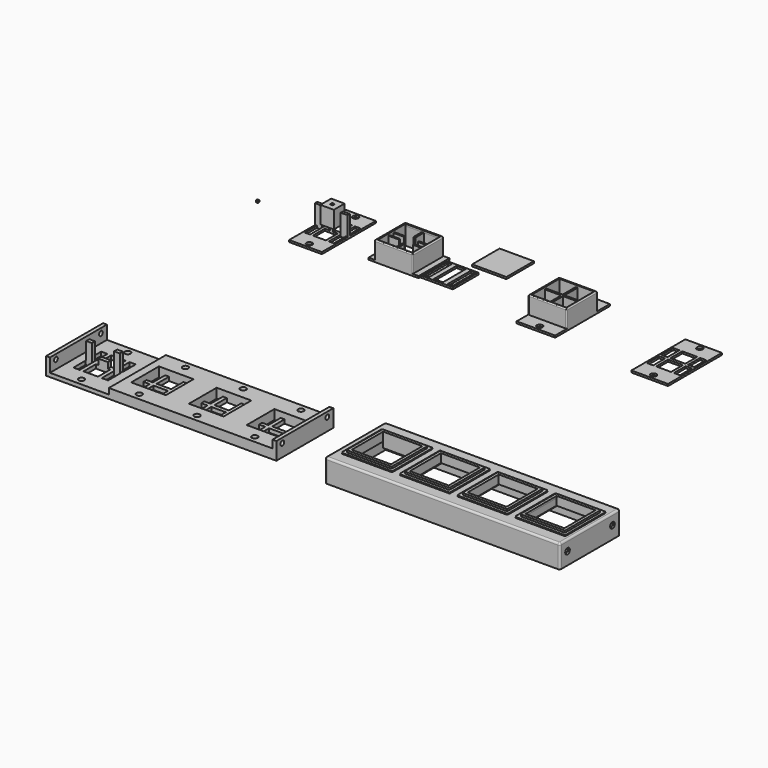
from build123d import *

# Parameters (mm, degrees)
F0_W          = 20
F0_H          = 20
F1_DEPTH      = 10
F2_T          = -1
F4_DEPTH      = 9
F5_W          = 20
F5_H          = 8
F5_R          = 1.5
F6_DEPTH      = 1
F7_W          = 19
F7_H          = 19
F7_H_2        = 8
F7_R          = 1.5
F8_DEPTH      = 1
F9_W          = 20
F9_H          = 20
F10_DEPTH     = 10
F11_W         = 3
F11_H         = 20
F11_W_2       = 20
F12_DEPTH     = 0.95
F13_T         = 1
F13_T3_DEPTH  = 22
F14_W         = 8.5
F14_H         = 0.8
F15_DEPTH     = 9
F17_DEPTH     = 9
F18_W         = 17
F18_H         = 8
F18_R         = 1.5
F18_H_2       = 19
F19_DEPTH     = 1
F20_W         = 1.5
F20_H         = 1.5
F21_DEPTH     = 3
F22_W         = 7
F22_H         = 7
F22_W_2       = 1.5
F22_H_2       = 1.5
F23_DEPTH     = 9
F24_W         = 1
F24_H         = 1
F25_DEPTH     = 1
F27_DEPTH     = 10
F28_W         = 0.9
F28_H         = 14.7
F28_W_2       = 2.5
F28_H_2       = 0.8
F28_H_3       = 6
F28_H_4       = 1.1
F29_DEPTH     = 1
F30_W         = 117
F30_H         = 37
F30_R         = 1.5
F31_DEPTH     = 1
F32_W         = 122
F32_H         = 39.2
F32_W_2       = 20.4
F32_H_2       = 20.4
F32_W_3       = 20.2
F32_H_3       = 20.2
F33_DEPTH     = 11
F34_W         = 120
F34_H         = 37.2
F35_DEPTH     = 8
F36_W         = 4
F36_H         = 18
F37_DEPTH     = 3
F39_W         = 3
F39_H         = 2
F40_DEPTH     = 9
F41_W         = 5
F41_H         = 2
F42_DEPTH     = 3
F43_R         = 1
F44_R         = 0.5
F44_2_R       = 0.5
F38_R         = 1.5
F45_DEPTH     = 3
F46_DEPTH     = 2
F47_W         = 2
F47_H         = 37
F48_DEPTH     = 7
F49_W         = 20.4
F49_H         = 8.4
F50_DEPTH     = 3
F51_R         = 1.5
F52_DEPTH     = 3
F54_R         = 1.5
F55_DEPTH     = 2
F56_W         = 3
F56_H         = 37.2
F57_DEPTH     = 1
F58_DEPTH     = 1
F59_W         = 2
F59_H         = 37
F60_DEPTH     = 4
F53_R         = 1.2
F61_DEPTH     = 269.2358512024
F62_DEPTH     = 3
F63_DEPTH     = 5
F46_FACE2_W   = 119
F46_FACE2_H   = 37
F46_FACE2_R   = 1.5
F46_FACE2_W_2 = 3.25
F46_FACE2_H_2 = 8
F46_FACE2_W_3 = 7.5
F64_DEPTH     = 1
F65_DEPTH     = 1
F66_DEPTH     = 2
F67_DEPTH     = 0.05
F68_W         = 20.4
F68_H         = 3
F68_W_2       = 20.2
F68_H_2       = 3.1
F69_DEPTH     = 0.5
F70_W         = 20.4
F70_H         = 1.5
F70_W_2       = 20.2
F71_DEPTH     = 1
F72_R         = 0.5
F73_W         = 18
F73_H         = 17.9999990673
F74_DEPTH     = 1
F75_W         = 17.8
F75_H         = 17.8
F76_DEPTH     = 1
F77_W         = 18
F77_H         = 18
F78_DEPTH     = 1


# Not quite as in the source:
# - a shell that OpenCascade refuses in one call is made with other operations: the cavity is built on its own and cut out
# - a feature names something its author has since deleted; it is built from what else it names


with BuildPart() as f1:
    # F0 (on Top) → F1 (new body)
    with BuildSketch(Plane.XY):
        Rectangle(F0_W, F0_H)
    extrude(amount=F1_DEPTH)

    # F2
    f2_openings = [f1.faces().sort_by_distance(p)[0] for p in [
        (0, 0, 0),
    ]]
    offset(amount=F2_T, openings=f2_openings)

    # F3 (on Top) → F4 (join)
    with BuildSketch(Plane.XY):
        Polygon((-0.5, -9), (0.5, -9), (0.5, -0.5), (9, -0.5), (9, 0.5), (0.5, 0.5), (0.5, 9), (-0.5, 9), (-0.5, 0.5), (-9, 0.5), (-9, -0.5), (-0.5, -0.5), align=None)
    extrude(amount=F4_DEPTH)

    # F5 (on Top) → F6 (join)
    with BuildSketch(Plane.XY):
        with Locations((0, -13.5)):
            Rectangle(F5_W, F5_H)
        with Locations((0, -15)):
            Circle(F5_R, mode=Mode.SUBTRACT)
        with Locations((0, 14)):
            Rectangle(F5_W, F5_H)
        with Locations((0, 15)):
            Circle(F5_R, mode=Mode.SUBTRACT)
    extrude(amount=F6_DEPTH)

    # F44
    f44_edges = [f1.edges().sort_by_distance(p)[0] for p in [
        (-10, -10, 5.5),
        (0, -10, 10),
        (10, -10, 5.5),
        (-10, 0, 10),
        (-10, 10, 5.5),
        (0, 10, 10),
        (10, 10, 5.5),
        (10, 0, 10),
    ]]
    fillet(f44_edges, radius=F44_R)

    # F77 (on face) → F78 (cut)
    with BuildSketch(Plane.XY.offset(10)):
        Rectangle(F77_W, F77_H)
    extrude(amount=-F78_DEPTH, mode=Mode.SUBTRACT)


with BuildPart() as f8:
    # F7 (on Top) → F8 (new body)
    with BuildSketch(Plane.XY):
        with Locations((62.8032131791, -4.6075988114)):
            Rectangle(F7_W, F7_H)
        Polygon((54.3032131791, -3.8575988114), (54.3032131791, 3.8924011886), (57.4282131791, 3.8924011886), (58.9282131791, 3.8924011886), (66.6782131791, 3.8924011886), (68.1782131791, 3.8924011886), (71.3032131791, 3.8924011886), (71.3032131791, -3.8575988114), (71.3032131791, -5.3575988114), (71.3032131791, -13.1075988114), (68.1782131791, -13.1075988114), (66.6782131791, -13.1075988114), (58.9282131791, -13.1075988114), (57.4282131791, -13.1075988114), (54.3032131791, -13.1075988114), (54.3032131791, -5.3575988114), align=None, mode=Mode.SUBTRACT)
        with Locations((62.8032131791, 8.8924011886)):
            Rectangle(F7_W, F7_H_2)
        with Locations((62.8032131791, 10.3924011886)):
            Circle(F7_R, mode=Mode.SUBTRACT)
        with Locations((62.8032131791, -18.1075988114)):
            Rectangle(F7_W, F7_H_2)
        with Locations((62.8032131791, -19.6075988114)):
            Circle(F7_R, mode=Mode.SUBTRACT)
        Polygon((58.9282131791, 3.8924011886), (57.4282131791, 3.8924011886), (57.4282131791, -3.8575988114), (54.3032131791, -3.8575988114), (54.3032131791, -5.3575988114), (57.4282131791, -5.3575988114), (57.4282131791, -13.1075988114), (58.9282131791, -13.1075988114), (58.9282131791, -5.3575988114), (66.6782131791, -5.3575988114), (66.6782131791, -13.1075988114), (68.1782131791, -13.1075988114), (68.1782131791, -5.3575988114), (71.3032131791, -5.3575988114), (71.3032131791, -3.8575988114), (68.1782131791, -3.8575988114), (68.1782131791, 3.8924011886), (66.6782131791, 3.8924011886), (66.6782131791, -3.8575988114), (58.9282131791, -3.8575988114), align=None)
    extrude(amount=F8_DEPTH)


with BuildPart() as f10:
    # F9 (on Top) → F10 (new body)
    with BuildSketch(Plane.XY):
        with Locations((-78.8846665621, -1.3073290847)):
            Rectangle(F9_W, F9_H)
    extrude(amount=F10_DEPTH)

    # F11 (on face) → F12 (join)
    with BuildSketch(Plane(origin=(0, 0, 0), x_dir=(1, 0, 0), z_dir=(0, 0, -1))):
        with Locations((-90.3846665621, 1.3073290847)):
            Rectangle(F11_W, F11_H)
        with Locations((-78.8846665621, 1.3073290847)):
            Rectangle(F11_W_2, F11_H)
        with Locations((-67.3846665621, 1.3073290847)):
            Rectangle(F11_W, F11_H)
    extrude(amount=-F12_DEPTH)

    # F13: shell of thickness 1, made by hand


with BuildPart() as f13_core1:
    # F13_t2: copy of F10
    add(f10.part)

    # the walls: a layer under each face that stays
    f13_faces = [f13_core1.faces().sort_by_distance(p)[0] for p in [
        (-78.8846665621, 8.6926709153, 5),
        (-91.8846665621, -1.3073290847, 0.475),
        (-78.8846665621, -11.3073290847, 5),
        (-90.3846665621, -1.3073290847, 0.95),
        (-88.8846665621, -1.3073290847, 5.475),
        (-78.8846665621, -1.3073290847, 10),
        (-68.8846665621, -1.3073290847, 5.475),
        (-67.3846665621, -1.3073290847, 0.95),
        (-65.8846665621, -1.3073290847, 0.475),
    ]]
    thicken(f13_faces, amount=-F13_T, mode=Mode.SUBTRACT)

    # F13_s4 → F13_t3 (cut)
    with BuildSketch(Plane.XZ.offset(-9.6926709153)):
        Polygon((-88.8946665621, 0.96), (-88.8846665621, -0.05), (-87.8846665621, -0.05), (-87.8846665621, 0.95), align=None)
        Polygon((-68.8746665621, 0.96), (-69.8846665621, 0.95), (-69.8846665621, -0.05), (-68.8846665621, -0.05), align=None)
    extrude(amount=F13_T3_DEPTH, mode=Mode.SUBTRACT)


with BuildPart() as f10_1:
    add(f10.part)

    # what is left inside the walls is the cavity
    f13_cavity = [f13_core1.part.solids().sort_by_distance(p)[0] for p in [
        (-78.884667, -4.307329, 0.01),
    ]]
    add(f13_cavity, mode=Mode.SUBTRACT)

    # F14 (on Top) → F15 (join)
    with BuildSketch(Plane.XY):
        Polygon((-78.3846665621, 7.6926709153), (-79.3846665621, 7.6926709153), (-79.3846665621, 0.6926709153), (-79.3846665621, -0.1073290847), (-79.3846665621, -2.5073290847), (-79.3846665621, -3.3073290847), (-79.3846665621, -10.3073290847), (-78.3846665621, -10.3073290847), (-78.3846665621, -3.3073290847), (-78.3846665621, -2.5073290847), (-78.3846665621, -0.1073290847), (-78.3846665621, 0.6926709153), align=None)
        with Locations((-83.6346665621, -2.9073290847)):
            Rectangle(F14_W, F14_H)
        with Locations((-83.6346665621, 0.2926709153)):
            Rectangle(F14_W, F14_H)
        with Locations((-74.1346665621, 0.2926709153)):
            Rectangle(F14_W, F14_H)
        with Locations((-74.1346665621, -2.9073290847)):
            Rectangle(F14_W, F14_H)
    extrude(amount=F15_DEPTH)

    # F16 (on face) → F17 (cut)
    with BuildSketch(Plane(origin=(0, 0, 0), x_dir=(1, 0, 0), z_dir=(0, 0, -1))):
        Polygon((-79.3846665621, -2.2926709153), (-78.3846665621, -2.2926709153), (-78.3846665621, -0.6926709153), (-75.2846665621, -0.6926709153), (-75.2846665621, 0.1073290847), (-78.3846665621, 0.1073290847), (-78.3846665621, 2.5073290847), (-75.2846665621, 2.5073290847), (-75.2846665621, 3.3073290847), (-78.3846665621, 3.3073290847), (-78.3846665621, 4.9073290847), (-79.3846665621, 4.9073290847), (-79.3846665621, 3.3073290847), (-82.4846665621, 3.3073290847), (-82.4846665621, 2.5073290847), (-79.3846665621, 2.5073290847), (-79.3846665621, 0.1073290847), (-82.4846665621, 0.1073290847), (-82.4846665621, -0.6926709153), (-79.3846665621, -0.6926709153), align=None)
    extrude(amount=-F17_DEPTH, mode=Mode.SUBTRACT)

    # F44#2
    f44_2_edges = [f10_1.edges().sort_by_distance(p)[0] for p in [
        (-68.884667, -11.307329, 5.475),
        (-78.884667, -11.307329, 10),
        (-68.884667, -1.307329, 10),
        (-68.884667, 8.692671, 5.475),
        (-78.884667, 8.692671, 10),
        (-88.884667, 8.692671, 5.475),
        (-88.884667, -1.307329, 10),
        (-88.884667, -11.307329, 5.475),
    ]]
    fillet(f44_2_edges, radius=F44_2_R)

    # F67 (add): faces of the model
    f67_faces = [f10_1.faces().sort_by_distance(p)[0] for p in [
        (-90.3817894545, -1.3073290847, 0.95),
        (-67.3875436696, -1.3073290847, 0.95),
    ]]
    extrude(f67_faces, amount=F67_DEPTH)

    # F73 (on face) → F74 (cut)
    with BuildSketch(Plane.XY.offset(10)):
        with Locations((-78.8846665621, -1.3073295511)):
            Rectangle(F73_W, F73_H)
    extrude(amount=-F74_DEPTH, mode=Mode.SUBTRACT)


with BuildPart() as f19:
    # F18 (on Top) → F19 (new body)
    with BuildSketch(Plane.XY):
        with Locations((-118.1940851788, 11.6607970074)):
            Rectangle(F18_W, F18_H)
        with Locations((-118.1940851788, 13.1607970074)):
            Circle(F18_R, mode=Mode.SUBTRACT)
        with Locations((-118.1940851788, -15.3392029926)):
            Rectangle(F18_W, F18_H)
        with Locations((-118.1940851788, -16.8392029926)):
            Circle(F18_R, mode=Mode.SUBTRACT)
        with Locations((-118.1940851788, -1.8392029926)):
            Rectangle(F18_W, F18_H_2)
        Polygon((-125.6940851788, -1.0892029926), (-125.6940851788, 6.6607970074), (-123.0690851788, 6.6607970074), (-121.5690851788, 6.6607970074), (-114.8190851788, 6.6607970074), (-113.3190851788, 6.6607970074), (-110.6940851788, 6.6607970074), (-110.6940851788, -1.0892029926), (-110.6940851788, -2.5892029926), (-110.6940851788, -10.3392029926), (-113.3190851788, -10.3392029926), (-114.8190851788, -10.3392029926), (-121.5690851788, -10.3392029926), (-123.0690851788, -10.3392029926), (-125.6940851788, -10.3392029926), (-125.6940851788, -2.5892029926), align=None, mode=Mode.SUBTRACT)
        Polygon((-121.5690851788, 6.6607970074), (-123.0690851788, 6.6607970074), (-123.0690851788, -1.0892029926), (-125.6940851788, -1.0892029926), (-125.6940851788, -2.5892029926), (-123.0690851788, -2.5892029926), (-123.0690851788, -10.3392029926), (-121.5690851788, -10.3392029926), (-121.5690851788, -2.5892029926), (-114.8190851788, -2.5892029926), (-114.8190851788, -10.3392029926), (-113.3190851788, -10.3392029926), (-113.3190851788, -2.5892029926), (-110.6940851788, -2.5892029926), (-110.6940851788, -1.0892029926), (-113.3190851788, -1.0892029926), (-113.3190851788, 6.6607970074), (-114.8190851788, 6.6607970074), (-114.8190851788, -1.0892029926), (-121.5690851788, -1.0892029926), align=None)
    extrude(amount=F19_DEPTH)

    # F20 (on face) → F21 (join)
    with BuildSketch(Plane.XY.offset(1)):
        with Locations((-118.1940851788, -1.8392029926)):
            Rectangle(F20_W, F20_H)
    extrude(amount=F21_DEPTH)

    # F26 (on face) → F27 (join)
    with BuildSketch(Plane.XY.offset(1)):
        Polygon((-109.6940851788, -2.5892029926), (-109.6940851788, -1.0892029926), (-110.6940851788, -1.0892029926), (-113.3190851788, -1.0892029926), (-113.3190851788, -2.5892029926), (-110.6940851788, -2.5892029926), align=None)
        Polygon((-125.6940851788, -1.0892029926), (-126.6940851788, -1.0892029926), (-126.6940851788, -2.5892029926), (-125.6940851788, -2.5892029926), (-123.0690851788, -2.5892029926), (-123.0690851788, -1.0892029926), align=None)
    extrude(amount=F27_DEPTH)


with BuildPart() as f23:
    # F22 (on face) → F23 (new body)
    with BuildSketch(Plane.XY.offset(4)):
        with Locations((-118.1940851788, -1.8392029926)):
            Rectangle(F22_W, F22_H)
        with Locations((-118.1940851788, -1.8392029926)):
            Rectangle(F22_W_2, F22_H_2, mode=Mode.SUBTRACT)
    extrude(amount=F23_DEPTH)


with BuildPart() as f25:
    # F24 (on Top) → F25 (new body)
    with BuildSketch(Plane.XY):
        with Locations((-158.5527062416, 0)):
            Rectangle(F24_W, F24_H)
    extrude(amount=F25_DEPTH)


with BuildPart() as f29:
    # F28 (on Top) → F29 (new body)
    with BuildSketch(Plane.XY):
        Polygon((-64.4713718057, -9.4157041669), (-65.3713718057, -9.4157041669), (-65.3713718057, -10.3157041669), (-54.7713718057, -10.3157041669), (-52.2713718057, -10.3157041669), (-48.8713718057, -10.3157041669), (-48.8713718057, -9.4157041669), (-49.7713718057, -9.4157041669), (-52.2713718057, -9.4157041669), (-54.7713718057, -9.4157041669), (-59.4713718057, -9.4157041669), (-61.9713718057, -9.4157041669), align=None)
        with Locations((-64.9213718057, -2.0657041669)):
            Rectangle(F28_W, F28_H)
        Polygon((-48.8713718057, 6.1842958331), (-65.3713718057, 6.1842958331), (-65.3713718057, 5.2842958331), (-64.4713718057, 5.2842958331), (-61.9713718057, 5.2842958331), (-59.4713718057, 5.2842958331), (-54.7713718057, 5.2842958331), (-52.2713718057, 5.2842958331), (-49.7713718057, 5.2842958331), (-48.8713718057, 5.2842958331), align=None)
        with Locations((-49.3213718057, -2.0657041669)):
            Rectangle(F28_W, F28_H)
        with Locations((-53.5213718057, 4.8842958331)):
            Rectangle(F28_W_2, F28_H_2)
        with Locations((-53.5213718057, 1.4842958331)):
            Rectangle(F28_W_2, F28_H_3)
        with Locations((-53.5213718057, -2.0657041669)):
            Rectangle(F28_W_2, F28_H_4)
        with Locations((-53.5213718057, -5.6157041669)):
            Rectangle(F28_W_2, F28_H_3)
        with Locations((-53.5213718057, -9.0157041669)):
            Rectangle(F28_W_2, F28_H_2)
        with Locations((-60.7213718057, 4.8842958331)):
            Rectangle(F28_W_2, F28_H_2)
        with Locations((-60.7213718057, 1.4842958331)):
            Rectangle(F28_W_2, F28_H_3)
        with Locations((-60.7213718057, -2.0657041669)):
            Rectangle(F28_W_2, F28_H_4)
        with Locations((-60.7213718057, -5.6157041669)):
            Rectangle(F28_W_2, F28_H_3)
        with Locations((-60.7213718057, -9.0157041669)):
            Rectangle(F28_W_2, F28_H_2)
    extrude(amount=F29_DEPTH)


with BuildPart() as f31:
    # F30 (on Top) → F31 (new body)
    with BuildSketch(Plane.XY):
        with Locations((-71.0754835367, -152.5580135584)):
            Rectangle(F30_W, F30_H)
        with Locations((-115.9754835367, -167.5580135584)):
            Circle(F30_R, mode=Mode.SUBTRACT)
        with Locations((-85.9754835367, -167.5580135584)):
            Circle(F30_R, mode=Mode.SUBTRACT)
        Polygon((-124.9754835367, -151.5580135584), (-124.9754835367, -143.5580135584), (-121.7254835367, -143.5580135584), (-119.7254835367, -143.5580135584), (-112.2254835367, -143.5580135584), (-110.2254835367, -143.5580135584), (-106.9754835367, -143.5580135584), (-106.9754835367, -151.5580135584), (-106.9754835367, -153.5580135584), (-106.9754835367, -161.5580135584), (-110.2254835367, -161.5580135584), (-112.2254835367, -161.5580135584), (-119.7254835367, -161.5580135584), (-121.7254835367, -161.5580135584), (-124.9754835367, -161.5580135584), (-124.9754835367, -153.5580135584), align=None, mode=Mode.SUBTRACT)
        Polygon((-94.9754835367, -151.5580135584), (-94.9754835367, -143.5580135584), (-91.7254835367, -143.5580135584), (-89.7254835367, -143.5580135584), (-82.2254835367, -143.5580135584), (-80.2254835367, -143.5580135584), (-76.9754835367, -143.5580135584), (-76.9754835367, -151.5580135584), (-76.9754835367, -153.5580135584), (-76.9754835367, -161.5580135584), (-80.2254835367, -161.5580135584), (-82.2254835367, -161.5580135584), (-89.7254835367, -161.5580135584), (-91.7254835367, -161.5580135584), (-94.9754835367, -161.5580135584), (-94.9754835367, -153.5580135584), align=None, mode=Mode.SUBTRACT)
        with Locations((-55.9754835367, -167.5580135584)):
            Circle(F30_R, mode=Mode.SUBTRACT)
        with Locations((-25.9754835367, -167.5580135584)):
            Circle(F30_R, mode=Mode.SUBTRACT)
        Polygon((-64.9754835367, -151.5580135584), (-64.9754835367, -143.5580135584), (-61.7254835367, -143.5580135584), (-59.7254835367, -143.5580135584), (-52.2254835367, -143.5580135584), (-50.2254835367, -143.5580135584), (-46.9754835367, -143.5580135584), (-46.9754835367, -151.5580135584), (-46.9754835367, -153.5580135584), (-46.9754835367, -161.5580135584), (-47.9754835367, -161.5580135584), (-50.2254835367, -161.5580135584), (-52.2254835367, -161.5580135584), (-59.7254835367, -161.5580135584), (-61.7254835367, -161.5580135584), (-64.9754835367, -161.5580135584), (-64.9754835367, -153.5580135584), align=None, mode=Mode.SUBTRACT)
        Polygon((-34.9754835367, -151.5580135584), (-34.9754835367, -143.5580135584), (-31.7254835367, -143.5580135584), (-29.7254835367, -143.5580135584), (-22.2254835367, -143.5580135584), (-20.2254835367, -143.5580135584), (-16.9754835367, -143.5580135584), (-16.9754835367, -151.5580135584), (-16.9754835367, -153.5580135584), (-16.9754835367, -161.5580135584), (-17.9754835367, -161.5580135584), (-20.2254835367, -161.5580135584), (-22.2254835367, -161.5580135584), (-29.7254835367, -161.5580135584), (-31.7254835367, -161.5580135584), (-34.9754835367, -161.5580135584), (-34.9754835367, -153.5580135584), align=None, mode=Mode.SUBTRACT)
        with Locations((-115.9754835367, -137.5580135584)):
            Circle(F30_R, mode=Mode.SUBTRACT)
        with Locations((-85.9754835367, -137.5580135584)):
            Circle(F30_R, mode=Mode.SUBTRACT)
        with Locations((-55.9754835367, -137.5580135584)):
            Circle(F30_R, mode=Mode.SUBTRACT)
        with Locations((-25.9754835367, -137.5580135584)):
            Circle(F30_R, mode=Mode.SUBTRACT)
        Polygon((-119.7254835367, -143.5580135584), (-121.7254835367, -143.5580135584), (-121.7254835367, -151.5580135584), (-124.9754835367, -151.5580135584), (-124.9754835367, -153.5580135584), (-121.7254835367, -153.5580135584), (-121.7254835367, -161.5580135584), (-119.7254835367, -161.5580135584), (-119.7254835367, -153.5580135584), (-112.2254835367, -153.5580135584), (-112.2254835367, -161.5580135584), (-110.2254835367, -161.5580135584), (-110.2254835367, -153.5580135584), (-106.9754835367, -153.5580135584), (-106.9754835367, -151.5580135584), (-110.2254835367, -151.5580135584), (-110.2254835367, -143.5580135584), (-112.2254835367, -143.5580135584), (-112.2254835367, -151.5580135584), (-119.7254835367, -151.5580135584), align=None)
        Polygon((-89.7254835367, -143.5580135584), (-91.7254835367, -143.5580135584), (-91.7254835367, -151.5580135584), (-94.9754835367, -151.5580135584), (-94.9754835367, -153.5580135584), (-91.7254835367, -153.5580135584), (-91.7254835367, -161.5580135584), (-89.7254835367, -161.5580135584), (-89.7254835367, -153.5580135584), (-82.2254835367, -153.5580135584), (-82.2254835367, -161.5580135584), (-80.2254835367, -161.5580135584), (-80.2254835367, -153.5580135584), (-76.9754835367, -153.5580135584), (-76.9754835367, -151.5580135584), (-80.2254835367, -151.5580135584), (-80.2254835367, -143.5580135584), (-82.2254835367, -143.5580135584), (-82.2254835367, -151.5580135584), (-89.7254835367, -151.5580135584), align=None)
        Polygon((-59.7254835367, -143.5580135584), (-61.7254835367, -143.5580135584), (-61.7254835367, -151.5580135584), (-64.9754835367, -151.5580135584), (-64.9754835367, -153.5580135584), (-61.7254835367, -153.5580135584), (-61.7254835367, -161.5580135584), (-59.7254835367, -161.5580135584), (-59.7254835367, -153.5580135584), (-52.2254835367, -153.5580135584), (-52.2254835367, -161.5580135584), (-50.2254835367, -161.5580135584), (-50.2254835367, -153.5580135584), (-46.9754835367, -153.5580135584), (-46.9754835367, -151.5580135584), (-50.2254835367, -151.5580135584), (-50.2254835367, -143.5580135584), (-52.2254835367, -143.5580135584), (-52.2254835367, -151.5580135584), (-59.7254835367, -151.5580135584), align=None)
        Polygon((-29.7254835367, -143.5580135584), (-31.7254835367, -143.5580135584), (-31.7254835367, -151.5580135584), (-34.9754835367, -151.5580135584), (-34.9754835367, -153.5580135584), (-31.7254835367, -153.5580135584), (-31.7254835367, -161.5580135584), (-29.7254835367, -161.5580135584), (-29.7254835367, -153.5580135584), (-22.2254835367, -153.5580135584), (-22.2254835367, -161.5580135584), (-20.2254835367, -161.5580135584), (-20.2254835367, -153.5580135584), (-16.9754835367, -153.5580135584), (-16.9754835367, -151.5580135584), (-20.2254835367, -151.5580135584), (-20.2254835367, -143.5580135584), (-22.2254835367, -143.5580135584), (-22.2254835367, -151.5580135584), (-29.7254835367, -151.5580135584), align=None)
    extrude(amount=F31_DEPTH)

    # F36 (on face) → F37 (join)
    with BuildSketch(Plane.XY.offset(1)):
        with Locations((-96.9754835367, -152.5580135584)):
            Rectangle(F36_W, F36_H)
        with Locations((-74.9754835367, -152.5580135584)):
            Rectangle(F36_W, F36_H)
        with Locations((-66.9754835367, -152.5580135584)):
            Rectangle(F36_W, F36_H)
        with Locations((-44.9754835367, -152.5580135584)):
            Rectangle(F36_W, F36_H)
        with Locations((-36.9754835367, -152.5580135584)):
            Rectangle(F36_W, F36_H)
        with Locations((-14.9754835367, -152.5580135584)):
            Rectangle(F36_W, F36_H)
    extrude(amount=F37_DEPTH)

    # F39 (on face) → F40 (join)
    with BuildSketch(Plane.XY.offset(1)):
        with Locations((-123.2254835367, -152.5580135584)):
            Rectangle(F39_W, F39_H)
        with Locations((-108.7254835367, -152.5580135584)):
            Rectangle(F39_W, F39_H)
    extrude(amount=F40_DEPTH)

    # F41 (on face) → F42 (join)
    with BuildSketch(Plane.XY.offset(1)):
        with Locations((-115.9754835367, -152.5580135584)):
            Rectangle(F41_W, F41_H)
    extrude(amount=F42_DEPTH)

    # F38 (on face) → F45 (join)
    with BuildSketch(Plane.XY.offset(1)):
        Polygon((-98.9754835367, -134.0580135584), (-98.9754835367, -143.5580135584), (-94.9754835367, -143.5580135584), (-91.7254835367, -143.5580135584), (-89.7254835367, -143.5580135584), (-82.2254835367, -143.5580135584), (-80.2254835367, -143.5580135584), (-76.9754835367, -143.5580135584), (-72.9754835367, -143.5580135584), (-72.9754835367, -134.0580135584), align=None)
        with Locations((-85.9754835367, -137.5580135584)):
            Circle(F38_R, mode=Mode.SUBTRACT)
        Polygon((-94.9754835367, -161.5580135584), (-98.9754835367, -161.5580135584), (-98.9754835367, -171.0580135584), (-72.9754835367, -171.0580135584), (-72.9754835367, -161.5580135584), (-76.9754835367, -161.5580135584), (-80.2254835367, -161.5580135584), (-82.2254835367, -161.5580135584), (-89.7254835367, -161.5580135584), (-91.7254835367, -161.5580135584), align=None)
        with Locations((-85.9754835367, -167.5580135584)):
            Circle(F38_R, mode=Mode.SUBTRACT)
        Polygon((-68.9754835367, -161.5580135584), (-68.9754835367, -171.0580135584), (-42.9754835367, -171.0580135584), (-42.9754835367, -161.5580135584), (-46.9754835367, -161.5580135584), (-50.2254835367, -161.5580135584), (-52.2254835367, -161.5580135584), (-59.7254835367, -161.5580135584), (-61.7254835367, -161.5580135584), (-64.9754835367, -161.5580135584), align=None)
        with Locations((-55.9754835367, -167.5580135584)):
            Circle(F38_R, mode=Mode.SUBTRACT)
        Polygon((-42.9754835367, -134.0580135584), (-68.9754835367, -134.0580135584), (-68.9754835367, -143.5580135584), (-64.9754835367, -143.5580135584), (-61.7254835367, -143.5580135584), (-59.7254835367, -143.5580135584), (-52.2254835367, -143.5580135584), (-50.2254835367, -143.5580135584), (-46.9754835367, -143.5580135584), (-42.9754835367, -143.5580135584), align=None)
        with Locations((-55.9754835367, -137.5580135584)):
            Circle(F38_R, mode=Mode.SUBTRACT)
        Polygon((-12.9754835367, -134.0580135584), (-38.9754835367, -134.0580135584), (-38.9754835367, -143.5580135584), (-34.9754835367, -143.5580135584), (-31.7254835367, -143.5580135584), (-29.7254835367, -143.5580135584), (-22.2254835367, -143.5580135584), (-20.2254835367, -143.5580135584), (-16.9754835367, -143.5580135584), (-12.9754835367, -143.5580135584), align=None)
        with Locations((-25.9754835367, -137.5580135584)):
            Circle(F38_R, mode=Mode.SUBTRACT)
        Polygon((-38.9754835367, -161.5580135584), (-38.9754835367, -171.0580135584), (-12.9754835367, -171.0580135584), (-12.9754835367, -161.5580135584), (-16.9754835367, -161.5580135584), (-20.2254835367, -161.5580135584), (-22.2254835367, -161.5580135584), (-29.7254835367, -161.5580135584), (-31.7254835367, -161.5580135584), (-34.9754835367, -161.5580135584), align=None)
        with Locations((-25.9754835367, -167.5580135584)):
            Circle(F38_R, mode=Mode.SUBTRACT)
    extrude(amount=F45_DEPTH)

    # F46 (add): a face of the model
    f46_faces = [f31.faces().sort_by_distance(p)[0] for p in [
        (-129.5754835367, -152.5580135584, 0.5),
    ]]
    extrude(f46_faces, amount=F46_DEPTH)

    # F47 (on face) → F48 (join)
    with BuildSketch(Plane.XY.offset(1)):
        with Locations((-130.5754835367, -152.5580135584)):
            Rectangle(F47_W, F47_H)
    extrude(amount=F48_DEPTH)

    # F58 (add): a face of the model
    f58_faces = [f31.faces().sort_by_distance(p)[0] for p in [
        (-12.9754835367, -152.5580135584, 2.5),
    ]]
    extrude(f58_faces, amount=F58_DEPTH)

    # F59 (on face) → F60 (join)
    with BuildSketch(Plane.XY.offset(4)):
        with Locations((-12.9754835367, -152.5580135584)):
            Rectangle(F59_W, F59_H)
    extrude(amount=F60_DEPTH)

    # F53 (on face) → F61 (cut, through all)
    with BuildSketch(Plane(origin=(-131.5754835367, 0, 0), x_dir=(0, -1, 0), z_dir=(-1, 0, 0))):
        with Locations((137.9580135584, 5.5)):
            Circle(F53_R)
        with Locations((167.1580135584, 5.5)):
            Circle(F53_R)
    extrude(amount=-F61_DEPTH, mode=Mode.SUBTRACT)

    # F63 (add): faces of the model
    f63_faces = [f31.faces().sort_by_distance(p)[0] for p in [
        (-72.9754835367, -152.5580135584, 2.5),
        (-42.9754835367, -152.5580135584, 2.5),
    ]]
    extrude(f63_faces, amount=F63_DEPTH)

    # F30 (on Top) + F46_face2 (on face) → F64 (join)
    with BuildSketch(Plane.XY):
        with Locations((-71.0754835367, -152.5580135584)):
            Rectangle(F30_W, F30_H)
        with Locations((-115.9754835367, -167.5580135584)):
            Circle(F30_R, mode=Mode.SUBTRACT)
        with Locations((-85.9754835367, -167.5580135584)):
            Circle(F30_R, mode=Mode.SUBTRACT)
        Polygon((-124.9754835367, -151.5580135584), (-124.9754835367, -143.5580135584), (-121.7254835367, -143.5580135584), (-119.7254835367, -143.5580135584), (-112.2254835367, -143.5580135584), (-110.2254835367, -143.5580135584), (-106.9754835367, -143.5580135584), (-106.9754835367, -151.5580135584), (-106.9754835367, -153.5580135584), (-106.9754835367, -161.5580135584), (-110.2254835367, -161.5580135584), (-112.2254835367, -161.5580135584), (-119.7254835367, -161.5580135584), (-121.7254835367, -161.5580135584), (-124.9754835367, -161.5580135584), (-124.9754835367, -153.5580135584), align=None, mode=Mode.SUBTRACT)
        Polygon((-94.9754835367, -151.5580135584), (-94.9754835367, -143.5580135584), (-91.7254835367, -143.5580135584), (-89.7254835367, -143.5580135584), (-82.2254835367, -143.5580135584), (-80.2254835367, -143.5580135584), (-76.9754835367, -143.5580135584), (-76.9754835367, -151.5580135584), (-76.9754835367, -153.5580135584), (-76.9754835367, -161.5580135584), (-80.2254835367, -161.5580135584), (-82.2254835367, -161.5580135584), (-89.7254835367, -161.5580135584), (-91.7254835367, -161.5580135584), (-94.9754835367, -161.5580135584), (-94.9754835367, -153.5580135584), align=None, mode=Mode.SUBTRACT)
        with Locations((-55.9754835367, -167.5580135584)):
            Circle(F30_R, mode=Mode.SUBTRACT)
        with Locations((-25.9754835367, -167.5580135584)):
            Circle(F30_R, mode=Mode.SUBTRACT)
        Polygon((-64.9754835367, -151.5580135584), (-64.9754835367, -143.5580135584), (-61.7254835367, -143.5580135584), (-59.7254835367, -143.5580135584), (-52.2254835367, -143.5580135584), (-50.2254835367, -143.5580135584), (-46.9754835367, -143.5580135584), (-46.9754835367, -151.5580135584), (-46.9754835367, -153.5580135584), (-46.9754835367, -161.5580135584), (-47.9754835367, -161.5580135584), (-50.2254835367, -161.5580135584), (-52.2254835367, -161.5580135584), (-59.7254835367, -161.5580135584), (-61.7254835367, -161.5580135584), (-64.9754835367, -161.5580135584), (-64.9754835367, -153.5580135584), align=None, mode=Mode.SUBTRACT)
        Polygon((-34.9754835367, -151.5580135584), (-34.9754835367, -143.5580135584), (-31.7254835367, -143.5580135584), (-29.7254835367, -143.5580135584), (-22.2254835367, -143.5580135584), (-20.2254835367, -143.5580135584), (-16.9754835367, -143.5580135584), (-16.9754835367, -151.5580135584), (-16.9754835367, -153.5580135584), (-16.9754835367, -161.5580135584), (-17.9754835367, -161.5580135584), (-20.2254835367, -161.5580135584), (-22.2254835367, -161.5580135584), (-29.7254835367, -161.5580135584), (-31.7254835367, -161.5580135584), (-34.9754835367, -161.5580135584), (-34.9754835367, -153.5580135584), align=None, mode=Mode.SUBTRACT)
        with Locations((-115.9754835367, -137.5580135584)):
            Circle(F30_R, mode=Mode.SUBTRACT)
        with Locations((-85.9754835367, -137.5580135584)):
            Circle(F30_R, mode=Mode.SUBTRACT)
        with Locations((-55.9754835367, -137.5580135584)):
            Circle(F30_R, mode=Mode.SUBTRACT)
        with Locations((-25.9754835367, -137.5580135584)):
            Circle(F30_R, mode=Mode.SUBTRACT)
    with BuildSketch(Plane(origin=(-72.3791549796, -152.5580135584, 0), x_dir=(1, 0, 0), z_dir=(0, 0, -1))):
        with Locations((0.3036714428, 0)):
            Rectangle(F46_FACE2_W, F46_FACE2_H)
        with Locations((-43.5963285572, 15)):
            Circle(F46_FACE2_R, mode=Mode.SUBTRACT)
        with Locations((-13.5963285572, 15)):
            Circle(F46_FACE2_R, mode=Mode.SUBTRACT)
        with Locations((-36.2213285572, 5)):
            Rectangle(F46_FACE2_W_2, F46_FACE2_H_2, mode=Mode.SUBTRACT)
        with Locations((-43.5963285572, 5)):
            Rectangle(F46_FACE2_W_3, F46_FACE2_H_2, mode=Mode.SUBTRACT)
        with Locations((-50.9713285572, 5)):
            Rectangle(F46_FACE2_W_2, F46_FACE2_H_2, mode=Mode.SUBTRACT)
        with Locations((-50.9713285572, -5)):
            Rectangle(F46_FACE2_W_2, F46_FACE2_H_2, mode=Mode.SUBTRACT)
        with Locations((-43.5963285572, -5)):
            Rectangle(F46_FACE2_W_3, F46_FACE2_H_2, mode=Mode.SUBTRACT)
        with Locations((-36.2213285572, -5)):
            Rectangle(F46_FACE2_W_2, F46_FACE2_H_2, mode=Mode.SUBTRACT)
        with Locations((-6.2213285572, 5)):
            Rectangle(F46_FACE2_W_2, F46_FACE2_H_2, mode=Mode.SUBTRACT)
        with Locations((-13.5963285572, 5)):
            Rectangle(F46_FACE2_W_3, F46_FACE2_H_2, mode=Mode.SUBTRACT)
        with Locations((-20.9713285572, 5)):
            Rectangle(F46_FACE2_W_2, F46_FACE2_H_2, mode=Mode.SUBTRACT)
        with Locations((-20.9713285572, -5)):
            Rectangle(F46_FACE2_W_2, F46_FACE2_H_2, mode=Mode.SUBTRACT)
        with Locations((-13.5963285572, -5)):
            Rectangle(F46_FACE2_W_3, F46_FACE2_H_2, mode=Mode.SUBTRACT)
        with Locations((-6.2213285572, -5)):
            Rectangle(F46_FACE2_W_2, F46_FACE2_H_2, mode=Mode.SUBTRACT)
        with Locations((16.4036714428, 15)):
            Circle(F46_FACE2_R, mode=Mode.SUBTRACT)
        with Locations((46.4036714428, 15)):
            Circle(F46_FACE2_R, mode=Mode.SUBTRACT)
        with Locations((23.7786714428, 5)):
            Rectangle(F46_FACE2_W_2, F46_FACE2_H_2, mode=Mode.SUBTRACT)
        with Locations((16.4036714428, 5)):
            Rectangle(F46_FACE2_W_3, F46_FACE2_H_2, mode=Mode.SUBTRACT)
        with Locations((9.0286714428, 5)):
            Rectangle(F46_FACE2_W_2, F46_FACE2_H_2, mode=Mode.SUBTRACT)
        with Locations((9.0286714428, -5)):
            Rectangle(F46_FACE2_W_2, F46_FACE2_H_2, mode=Mode.SUBTRACT)
        with Locations((16.4036714428, -5)):
            Rectangle(F46_FACE2_W_3, F46_FACE2_H_2, mode=Mode.SUBTRACT)
        with Locations((23.7786714428, -5)):
            Rectangle(F46_FACE2_W_2, F46_FACE2_H_2, mode=Mode.SUBTRACT)
        with Locations((53.7786714428, 5)):
            Rectangle(F46_FACE2_W_2, F46_FACE2_H_2, mode=Mode.SUBTRACT)
        with Locations((46.4036714428, 5)):
            Rectangle(F46_FACE2_W_3, F46_FACE2_H_2, mode=Mode.SUBTRACT)
        with Locations((39.0286714428, 5)):
            Rectangle(F46_FACE2_W_2, F46_FACE2_H_2, mode=Mode.SUBTRACT)
        with Locations((39.0286714428, -5)):
            Rectangle(F46_FACE2_W_2, F46_FACE2_H_2, mode=Mode.SUBTRACT)
        with Locations((46.4036714428, -5)):
            Rectangle(F46_FACE2_W_3, F46_FACE2_H_2, mode=Mode.SUBTRACT)
        with Locations((53.7786714428, -5)):
            Rectangle(F46_FACE2_W_2, F46_FACE2_H_2, mode=Mode.SUBTRACT)
        with Locations((-43.5963285572, -15)):
            Circle(F46_FACE2_R, mode=Mode.SUBTRACT)
        with Locations((-13.5963285572, -15)):
            Circle(F46_FACE2_R, mode=Mode.SUBTRACT)
        with Locations((16.4036714428, -15)):
            Circle(F46_FACE2_R, mode=Mode.SUBTRACT)
        with Locations((46.4036714428, -15)):
            Circle(F46_FACE2_R, mode=Mode.SUBTRACT)
    extrude(amount=-F64_DEPTH, dir=(0, 0, 1))

    # F66 (add): a face of the model
    f66_faces = [f31.faces().sort_by_distance(p)[0] for p in [
        (-12.2754835367, -152.5580135584, 1),
    ]]
    extrude(f66_faces, amount=F66_DEPTH)


with BuildPart() as f33:
    # F32 (on Top) → F33 (new body)
    with BuildSketch(Plane.XY):
        with Locations((76.6593676656, -154.4580135584)):
            Rectangle(F32_W, F32_H)
        with Locations((32.2593676656, -154.4580135584)):
            Rectangle(F32_W_2, F32_H_2, mode=Mode.SUBTRACT)
        with Locations((62.2593676656, -154.4580135584)):
            Rectangle(F32_W_3, F32_H_3, mode=Mode.SUBTRACT)
        with Locations((92.2593676656, -154.4580135584)):
            Rectangle(F32_W_3, F32_H_3, mode=Mode.SUBTRACT)
        with Locations((122.2593676656, -154.4580135584)):
            Rectangle(F32_W_3, F32_H_3, mode=Mode.SUBTRACT)
    extrude(amount=F33_DEPTH)

    # F34 (on face) → F35 (cut)
    with BuildSketch(Plane(origin=(0, 0, 0), x_dir=(1, 0, 0), z_dir=(0, 0, -1))):
        with Locations((76.6593676656, 154.4580135584)):
            Rectangle(F34_W, F34_H)
    extrude(amount=-F35_DEPTH, mode=Mode.SUBTRACT)

    # F43
    f43_edges = [f33.edges().sort_by_distance(p)[0] for p in [
        (15.659368, -134.858014, 5.5),
        (15.659368, -174.058014, 5.5),
        (137.659368, -174.058014, 5.5),
        (137.659368, -134.858014, 5.5),
        (76.659368, -174.058014, 11),
        (15.659368, -154.458014, 11),
        (76.659368, -134.858014, 11),
        (137.659368, -154.458014, 11),
    ]]
    fillet(f43_edges, radius=F43_R)

    # F49 (on face) → F50 (join)
    with BuildSketch(Plane(origin=(0, 0, 8), x_dir=(1, 0, 0), z_dir=(0, 0, -1))):
        with Locations((32.2593676656, 168.8580135584)):
            Rectangle(F49_W, F49_H)
        with Locations((32.2593676656, 140.0580135584)):
            Rectangle(F49_W, F49_H)
    extrude(amount=F50_DEPTH)

    # F51 (on face) → F52 (cut)
    with BuildSketch(Plane(origin=(15.6593676656, 0, 0), x_dir=(0, -1, 0), z_dir=(-1, 0, 0))):
        with Locations((139.8580135584, 5.5)):
            Circle(F51_R)
        with Locations((169.0580135584, 5.5)):
            Circle(F51_R)
    extrude(amount=-F52_DEPTH, mode=Mode.SUBTRACT)

    # F54 (on face) → F55 (cut)
    with BuildSketch(Plane.YZ.offset(137.6593676656)):
        with Locations((-169.0580135584, 5.5)):
            Circle(F54_R)
        with Locations((-139.8580135584, 5.5)):
            Circle(F54_R)
    extrude(amount=-F55_DEPTH, mode=Mode.SUBTRACT)

    # F56 (on face) → F57 (join)
    with BuildSketch(Plane(origin=(0, 0, 8), x_dir=(1, 0, 0), z_dir=(0, 0, -1))):
        with Locations((47.4593676656, 154.4580135584)):
            Rectangle(F56_W, F56_H)
        with Locations((77.3593676656, 154.4580135584)):
            Rectangle(F56_W, F56_H)
        with Locations((107.3593676656, 154.4580135584)):
            Rectangle(F56_W, F56_H)
    extrude(amount=F57_DEPTH)

    # F56 (on face) → F62 (join)
    with BuildSketch(Plane(origin=(0, 0, 8), x_dir=(1, 0, 0), z_dir=(0, 0, -1))):
        with Locations((47.4593676656, 154.4580135584)):
            Rectangle(F56_W, F56_H)
        with Locations((77.3593676656, 154.4580135584)):
            Rectangle(F56_W, F56_H)
        with Locations((107.3593676656, 154.4580135584)):
            Rectangle(F56_W, F56_H)
    extrude(amount=F62_DEPTH)

    # F65 (add): a face of the model
    f65_faces = [f33.faces().sort_by_distance(p)[0] for p in [
        (137.5312246206, -154.4580135584, 0),
    ]]
    extrude(f65_faces, amount=F65_DEPTH)

    # F68 (on face) → F69 (join)
    with BuildSketch(Plane.XY.offset(11)):
        with Locations((32.2593676656, -142.7580135584)):
            Rectangle(F68_W, F68_H)
        Polygon((22.0593676656, -164.6580135584), (22.0593676656, -144.2580135584), (22.0593676656, -141.2580135584), (19.0593676656, -141.2580135584), (19.0593676656, -167.6580135584), (22.0593676656, -167.6580135584), align=None)
        Polygon((42.4593676656, -141.2580135584), (42.4593676656, -144.2580135584), (42.4593676656, -164.6580135584), (42.4593676656, -167.6580135584), (45.4593676656, -167.6580135584), (45.4593676656, -141.2580135584), align=None)
        with Locations((32.2593676656, -166.1580135584)):
            Rectangle(F68_W, F68_H)
        with Locations((62.2593676656, -142.8080135584)):
            Rectangle(F68_W_2, F68_H_2)
        Polygon((52.1593676656, -164.5580135584), (52.1593676656, -144.3580135584), (52.1593676656, -141.2580135584), (49.1593676656, -141.2580135584), (49.1593676656, -167.6580135584), (52.1593676656, -167.6580135584), align=None)
        Polygon((72.3593676656, -141.2580135584), (72.3593676656, -144.3580135584), (72.3593676656, -164.5580135584), (72.3593676656, -167.6580135584), (75.3593676656, -167.6580135584), (75.3593676656, -141.2580135584), align=None)
        with Locations((62.2593676656, -166.1080135584)):
            Rectangle(F68_W_2, F68_H_2)
        with Locations((92.2593676656, -142.8080135584)):
            Rectangle(F68_W_2, F68_H_2)
        Polygon((82.1593676656, -164.5580135584), (82.1593676656, -144.3580135584), (82.1593676656, -141.2580135584), (79.1593676656, -141.2580135584), (79.1593676656, -167.6580135584), (82.1593676656, -167.6580135584), align=None)
        Polygon((102.3593676656, -141.2580135584), (102.3593676656, -144.3580135584), (102.3593676656, -164.5580135584), (102.3593676656, -167.6580135584), (105.3593676656, -167.6580135584), (105.3593676656, -141.2580135584), align=None)
        with Locations((92.2593676656, -166.1080135584)):
            Rectangle(F68_W_2, F68_H_2)
        with Locations((122.2593676656, -142.8080135584)):
            Rectangle(F68_W_2, F68_H_2)
        Polygon((112.1593676656, -164.5580135584), (112.1593676656, -144.3580135584), (112.1593676656, -141.2580135584), (109.1593676656, -141.2580135584), (109.1593676656, -167.6580135584), (112.1593676656, -167.6580135584), align=None)
        Polygon((132.3593676656, -141.2580135584), (132.3593676656, -144.3580135584), (132.3593676656, -164.5580135584), (132.3593676656, -167.6580135584), (135.3593676656, -167.6580135584), (135.3593676656, -141.2580135584), align=None)
        with Locations((122.2593676656, -166.1080135584)):
            Rectangle(F68_W_2, F68_H_2)
    extrude(amount=F69_DEPTH)

    # F70 (on face) → F71 (join)
    with BuildSketch(Plane.XY.offset(11.5)):
        with Locations((32.2593676656, -143.5080135584)):
            Rectangle(F70_W, F70_H)
        Polygon((22.0593676656, -164.6580135584), (22.0593676656, -144.2580135584), (22.0593676656, -142.7580135584), (20.5593676656, -142.7580135584), (20.5593676656, -166.1580135584), (22.0593676656, -166.1580135584), align=None)
        Polygon((42.4593676656, -142.7580135584), (42.4593676656, -144.2580135584), (42.4593676656, -164.6580135584), (42.4593676656, -166.1580135584), (43.9593676656, -166.1580135584), (43.9593676656, -142.7580135584), align=None)
        with Locations((32.2593676656, -165.4080135584)):
            Rectangle(F70_W, F70_H)
        Polygon((52.1593676656, -142.8580135584), (50.6593676656, -142.8580135584), (50.6593676656, -166.0580135584), (52.1593676656, -166.0580135584), (52.1593676656, -164.5580135584), (52.1593676656, -144.3580135584), align=None)
        with Locations((62.2593676656, -143.6080135584)):
            Rectangle(F70_W_2, F70_H)
        Polygon((73.8593676656, -142.8580135584), (72.3593676656, -142.8580135584), (72.3593676656, -144.3580135584), (72.3593676656, -164.5580135584), (72.3593676656, -166.0580135584), (73.8593676656, -166.0580135584), align=None)
        with Locations((62.2593676656, -165.3080135584)):
            Rectangle(F70_W_2, F70_H)
        Polygon((82.1593676656, -142.8580135584), (80.6593676656, -142.8580135584), (80.6593676656, -166.0580135584), (82.1593676656, -166.0580135584), (82.1593676656, -164.5580135584), (82.1593676656, -144.3580135584), align=None)
        with Locations((92.2593676656, -143.6080135584)):
            Rectangle(F70_W_2, F70_H)
        Polygon((103.8593676656, -142.8580135584), (102.3593676656, -142.8580135584), (102.3593676656, -144.3580135584), (102.3593676656, -164.5580135584), (102.3593676656, -166.0580135584), (103.8593676656, -166.0580135584), align=None)
        with Locations((92.2593676656, -165.3080135584)):
            Rectangle(F70_W_2, F70_H)
        Polygon((112.2593676656, -142.8580135584), (110.7593676656, -142.8580135584), (110.7593676656, -166.0580135584), (112.2593676656, -166.0580135584), (112.2593676656, -164.5580135584), (112.2593676656, -144.3580135584), align=None)
        with Locations((122.3593676656, -143.6080135584)):
            Rectangle(F70_W_2, F70_H)
        Polygon((133.9593676656, -142.8580135584), (132.4593676656, -142.8580135584), (132.4593676656, -144.3580135584), (132.4593676656, -164.5580135584), (132.4593676656, -166.0580135584), (133.9593676656, -166.0580135584), align=None)
        with Locations((122.3593676656, -165.3080135584)):
            Rectangle(F70_W_2, F70_H)
    extrude(amount=F71_DEPTH)

    # F72
    f72_edges = [f33.edges().sort_by_distance(p)[0] for p in [
        (19.059368, -141.258014, 11.25),
        (20.559368, -142.758014, 12),
        (19.059368, -167.658014, 11.25),
        (20.559368, -166.158014, 12),
        (43.959368, -166.158014, 12),
        (45.459368, -167.658014, 11.25),
        (43.959368, -142.758014, 12),
        (45.459368, -141.258014, 11.25),
        (49.159368, -141.258014, 11.25),
        (50.659368, -142.858014, 12),
        (50.659368, -166.058014, 12),
        (49.159368, -167.658014, 11.25),
        (73.859368, -166.058014, 12),
        (75.359368, -167.658014, 11.25),
        (73.859368, -142.858014, 12),
        (75.359368, -141.258014, 11.25),
        (79.159368, -141.258014, 11.25),
        (80.659368, -142.858014, 12),
        (79.159368, -167.658014, 11.25),
        (80.659368, -166.058014, 12),
        (103.859368, -166.058014, 12),
        (105.359368, -167.658014, 11.25),
        (103.859368, -142.858014, 12),
        (105.359368, -141.258014, 11.25),
        (109.159368, -141.258014, 11.25),
        (110.759368, -142.858014, 12),
        (109.159368, -167.658014, 11.25),
        (110.759368, -166.058014, 12),
        (133.959368, -166.058014, 12),
        (135.359368, -167.658014, 11.25),
        (133.959368, -142.858014, 12),
        (135.359368, -141.258014, 11.25),
    ]]
    fillet(f72_edges, radius=F72_R)


with BuildPart() as f76:
    # F75 (on Top) → F76 (new body)
    with BuildSketch(Plane.XY):
        with Locations((-46.4569205403, 19.1935256436)):
            Rectangle(F75_W, F75_H)
    extrude(amount=F76_DEPTH)


solid = Compound([f1.part, f8.part, f10_1.part, f19.part, f23.part, f25.part, f29.part, f31.part, f33.part, f76.part])
